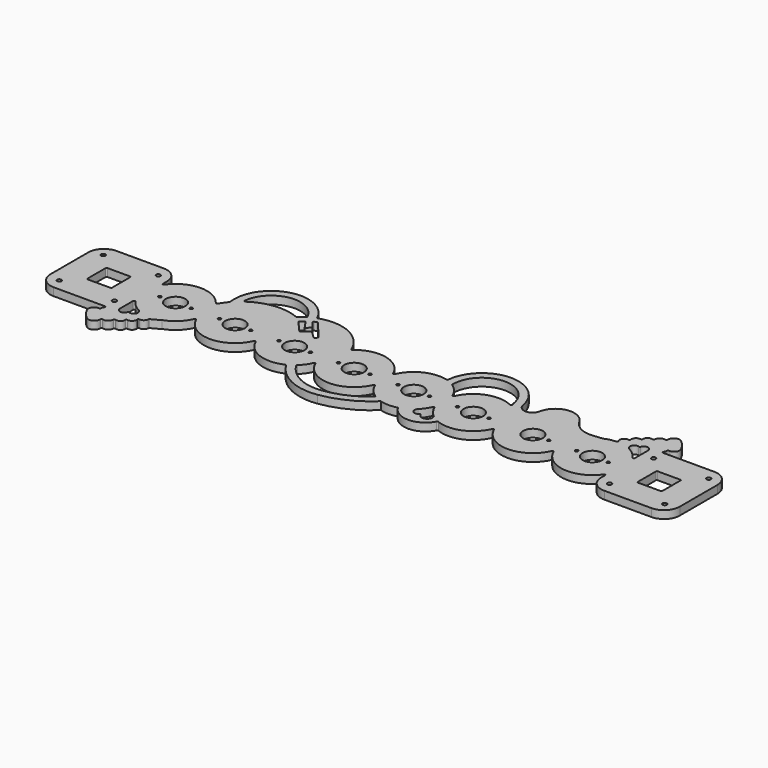
from build123d import *

# Parameters (mm, degrees)
F1_DEPTH  = 6.35
F2_R      = 25.4
F4_DEPTH  = 12.7
F6_DEPTH  = 12.7
F8_DEPTH  = 12.7
F10_DEPTH = 12.7
F12_DEPTH = 12.701
F14_DEPTH = 12.701
F16_D     = 6.7564
F18_D     = 31.75
F20_D     = 4.7625
F21_R     = 1.5875


# Not quite as in the source:
# - a feature names something its author has since deleted; it is built from what else it names


with BuildPart() as f1:
    # F0 (on Top) → F1 (new body, symmetric)
    with BuildSketch(Plane.XY):
        with BuildLine():
            Line((508, -63.5), (508, 63.5))
            Line((508, 63.5), (381, 63.5))
            Line((381, 63.5), (381, 24.5934442484))
            ThreePointArc((381, 24.5934442484), (385.7368884968, 12.7), (387.35, 0))
            ThreePointArc((387.35, 0), (385.7368884968, -12.7), (381, -24.5934442484))
            Line((381, -24.5934442484), (381, -63.5))
            Line((381, -63.5), (508, -63.5))
        make_face()
        with BuildLine():
            ThreePointArc((387.35, 0), (385.7368884968, 12.7), (381, 24.5934442484))
            Line((381, 24.5934442484), (381, 0))
            Line((381, 0), (387.35, 0))
        make_face()
        with BuildLine():
            Line((381, 0), (381, 24.5934442484))
            ThreePointArc((381, 24.5934442484), (332.0713380674, 50.6021895504), (288.4714285714, 16.4039924832))
            ThreePointArc((288.4714285714, 16.4039924832), (290.5078819786, 8.314101618), (291.1928571429, 0))
            ThreePointArc((291.1928571429, 0), (290.5078819786, -8.314101618), (288.4714285714, -16.4039924832))
            ThreePointArc((288.4714285714, -16.4039924832), (332.0713380674, -50.6021895504), (381, -24.5934442484))
            Line((381, -24.5934442484), (381, 0))
        make_face()
        with BuildLine():
            Line((387.35, 0), (381, 0))
            Line((381, 0), (381, -24.5934442484))
            ThreePointArc((381, -24.5934442484), (385.7368884968, -12.7), (387.35, 0))
        make_face()
        with BuildLine():
            ThreePointArc((288.4714285714, -16.4039924832), (285.75, 0), (288.4714285714, 16.4039924832))
            ThreePointArc((288.4714285714, 16.4039924832), (240.3928571429, 50.8), (192.3142857143, 16.4039924832))
            ThreePointArc((192.3142857143, 16.4039924832), (194.3507391214, 8.314101618), (195.0357142857, 0))
            ThreePointArc((195.0357142857, 0), (194.3507391214, -8.314101618), (192.3142857143, -16.4039924832))
            ThreePointArc((192.3142857143, -16.4039924832), (240.3928571429, -50.8), (288.4714285714, -16.4039924832))
        make_face()
        with BuildLine():
            ThreePointArc((291.1928571429, 0), (290.5078819786, 8.314101618), (288.4714285714, 16.4039924832))
            ThreePointArc((288.4714285714, 16.4039924832), (285.75, 0), (288.4714285714, -16.4039924832))
            ThreePointArc((288.4714285714, -16.4039924832), (290.5078819786, -8.314101618), (291.1928571429, 0))
        make_face()
        with BuildLine():
            ThreePointArc((192.3142857143, -16.4039924832), (189.5928571429, 0), (192.3142857143, 16.4039924832))
            ThreePointArc((192.3142857143, 16.4039924832), (144.2357142857, 50.8), (96.1571428571, 16.4039924832))
            ThreePointArc((96.1571428571, 16.4039924832), (98.1935962643, 8.314101618), (98.8785714286, 0))
            ThreePointArc((98.8785714286, 0), (98.1935962643, -8.314101618), (96.1571428571, -16.4039924832))
            ThreePointArc((96.1571428571, -16.4039924832), (144.2357142857, -50.8), (192.3142857143, -16.4039924832))
        make_face()
        with BuildLine():
            ThreePointArc((195.0357142857, 0), (194.3507391214, 8.314101618), (192.3142857143, 16.4039924832))
            ThreePointArc((192.3142857143, 16.4039924832), (189.5928571429, 0), (192.3142857143, -16.4039924832))
            ThreePointArc((192.3142857143, -16.4039924832), (194.3507391214, -8.314101618), (195.0357142857, 0))
        make_face()
        with BuildLine():
            ThreePointArc((96.1571428571, -16.4039924832), (93.4357142857, 0), (96.1571428571, 16.4039924832))
            ThreePointArc((96.1571428571, 16.4039924832), (48.0785714286, 50.8), (0, 16.4039924832))
            ThreePointArc((0, 16.4039924832), (2.0364534072, 8.314101618), (2.7214285714, 0))
            ThreePointArc((2.7214285714, 0), (2.0364534072, -8.314101618), (0, -16.4039924832))
            ThreePointArc((0, -16.4039924832), (48.0785714286, -50.8), (96.1571428571, -16.4039924832))
        make_face()
        with BuildLine():
            ThreePointArc((98.8785714286, 0), (98.1935962643, 8.314101618), (96.1571428571, 16.4039924832))
            ThreePointArc((96.1571428571, 16.4039924832), (93.4357142857, 0), (96.1571428571, -16.4039924832))
            ThreePointArc((96.1571428571, -16.4039924832), (98.1935962643, -8.314101618), (98.8785714286, 0))
        make_face()
        with BuildLine():
            ThreePointArc((0, -16.4039924832), (-2.7214285714, 0), (0, 16.4039924832))
            ThreePointArc((0, 16.4039924832), (-48.0785714286, 50.8), (-96.1571428571, 16.4039924832))
            ThreePointArc((-96.1571428571, 16.4039924832), (-94.12068945, 8.314101618), (-93.4357142857, 0))
            ThreePointArc((-93.4357142857, 0), (-94.12068945, -8.314101618), (-96.1571428571, -16.4039924832))
            ThreePointArc((-96.1571428571, -16.4039924832), (-48.0785714286, -50.8), (0, -16.4039924832))
        make_face()
        with BuildLine():
            ThreePointArc((2.7214285714, 0), (2.0364534072, 8.314101618), (0, 16.4039924832))
            ThreePointArc((0, 16.4039924832), (-2.7214285714, 0), (0, -16.4039924832))
            ThreePointArc((0, -16.4039924832), (2.0364534072, -8.314101618), (2.7214285714, 0))
        make_face()
        with BuildLine():
            ThreePointArc((-96.1571428571, -16.4039924832), (-98.8785714286, 0), (-96.1571428571, 16.4039924832))
            ThreePointArc((-96.1571428571, 16.4039924832), (-144.2357142857, 50.8), (-192.3142857143, 16.4039924832))
            ThreePointArc((-192.3142857143, 16.4039924832), (-190.2778323071, 8.314101618), (-189.5928571429, 0))
            ThreePointArc((-189.5928571429, 0), (-190.2778323071, -8.314101618), (-192.3142857143, -16.4039924832))
            ThreePointArc((-192.3142857143, -16.4039924832), (-144.2357142857, -50.8), (-96.1571428571, -16.4039924832))
        make_face()
        with BuildLine():
            ThreePointArc((-93.4357142857, 0), (-94.12068945, 8.314101618), (-96.1571428571, 16.4039924832))
            ThreePointArc((-96.1571428571, 16.4039924832), (-98.8785714286, 0), (-96.1571428571, -16.4039924832))
            ThreePointArc((-96.1571428571, -16.4039924832), (-94.12068945, -8.314101618), (-93.4357142857, 0))
        make_face()
        with BuildLine():
            ThreePointArc((-192.3142857143, -16.4039924832), (-195.0357142857, 0), (-192.3142857143, 16.4039924832))
            ThreePointArc((-192.3142857143, 16.4039924832), (-240.3928571429, 50.8), (-288.4714285714, 16.4039924832))
            ThreePointArc((-288.4714285714, 16.4039924832), (-286.4349751643, 8.314101618), (-285.75, 0))
            ThreePointArc((-285.75, 0), (-286.4349751643, -8.314101618), (-288.4714285714, -16.4039924832))
            ThreePointArc((-288.4714285714, -16.4039924832), (-240.3928571429, -50.8), (-192.3142857143, -16.4039924832))
        make_face()
        with BuildLine():
            ThreePointArc((-189.5928571429, 0), (-190.2778323071, 8.314101618), (-192.3142857143, 16.4039924832))
            ThreePointArc((-192.3142857143, 16.4039924832), (-195.0357142857, 0), (-192.3142857143, -16.4039924832))
            ThreePointArc((-192.3142857143, -16.4039924832), (-190.2778323071, -8.314101618), (-189.5928571429, 0))
        make_face()
        with BuildLine():
            ThreePointArc((-288.4714285714, -16.4039924832), (-291.1928571429, 0), (-288.4714285714, 16.4039924832))
            ThreePointArc((-288.4714285714, 16.4039924832), (-332.0713380674, 50.6021895504), (-381, 24.5934442484))
            Line((-381, 24.5934442484), (-381, 0))
            Line((-381, 0), (-381, -24.5934442484))
            ThreePointArc((-381, -24.5934442484), (-332.0713380674, -50.6021895504), (-288.4714285714, -16.4039924832))
        make_face()
        with BuildLine():
            ThreePointArc((-285.75, 0), (-286.4349751643, 8.314101618), (-288.4714285714, 16.4039924832))
            ThreePointArc((-288.4714285714, 16.4039924832), (-291.1928571429, 0), (-288.4714285714, -16.4039924832))
            ThreePointArc((-288.4714285714, -16.4039924832), (-286.4349751643, -8.314101618), (-285.75, 0))
        make_face()
        with BuildLine():
            ThreePointArc((-387.35, 0), (-385.7368884968, 12.7), (-381, 24.5934442484))
            Line((-381, 24.5934442484), (-381, 63.5))
            Line((-381, 63.5), (-508, 63.5))
            Line((-508, 63.5), (-508, -63.5))
            Line((-508, -63.5), (-381, -63.5))
            Line((-381, -63.5), (-381, -24.5934442484))
            ThreePointArc((-381, -24.5934442484), (-385.7368884968, -12.7), (-387.35, 0))
        make_face()
        with BuildLine():
            Line((-381, 0), (-381, 24.5934442484))
            ThreePointArc((-381, 24.5934442484), (-385.7368884968, 12.7), (-387.35, 0))
            Line((-387.35, 0), (-381, 0))
        make_face()
        with BuildLine():
            Line((-381, -24.5934442484), (-381, 0))
            Line((-381, 0), (-387.35, 0))
            ThreePointArc((-387.35, 0), (-385.7368884968, -12.7), (-381, -24.5934442484))
        make_face()
    extrude(amount=F1_DEPTH, both=True)

    # F2
    f2_edges = [f1.edges().sort_by_distance(p)[0] for p in [
        (508, -63.5, 0),
        (381, -63.5, 0),
        (508, 63.5, 0),
        (-508, -63.5, 0),
        (-508, 63.5, 0),
        (-381, 63.5, 0),
    ]]
    fillet(f2_edges, radius=F2_R)

    # F3 (on face) → F4 (join, through all)
    with BuildSketch(Plane.XY.offset(6.35)):
        with BuildLine():
            ThreePointArc((-367.2552444243, -56.6276222122), (-374.1276222122, -63.5), (-381, -56.6276222122))
            Line((-381, -56.6276222122), (-381, -63.5))
            Line((-381, -63.5), (-391.535417959, -63.5))
            Line((-391.535417959, -63.5), (-394.5178569695, -63.5))
            ThreePointArc((-394.5178569695, -63.5), (-399.2758099526, -67.1825538995), (-399.4201421738, -73.1974095106))
            ThreePointArc((-399.4201421738, -73.1974095106), (-409.2730898493, -75.0079193762), (-411.5812182426, -84.7563073039))
            ThreePointArc((-411.5812182426, -84.7563073039), (-405.652510141, -94.2560722227), (-397.9265391827, -102.3619025946))
            ThreePointArc((-397.9265391827, -102.3619025946), (-385.82556258, -103.1087125948), (-382.9926252365, -91.320335865))
            ThreePointArc((-382.9926252365, -91.320335865), (-371.9326843725, -91.8099168303), (-369.8217202848, -80.9422670357))
            ThreePointArc((-369.8217202848, -80.9422670357), (-359.9477437268, -83.4855580061), (-357.2103527895, -73.6636216957))
            ThreePointArc((-357.2103527895, -73.6636216957), (-347.2490954144, -72.7221806555), (-346.8697477111, -62.723728023))
            ThreePointArc((-346.8697477111, -62.723728023), (-336.1545012002, -61.4010311927), (-338.0772106471, -50.7770383898))
            ThreePointArc((-338.0772106471, -50.7770383898), (-349.2473790256, -49.187565155), (-359.791204809, -45.1717433694))
            ThreePointArc((-359.791204809, -45.1717433694), (-357.1773168684, -55.0343377987), (-367.2552444243, -56.6276222122))
        make_face()
        with BuildLine():
            ThreePointArc((-369.9145615101, -80.7840153575), (-369.867712705, -80.8628899897), (-369.8217202848, -80.9422670357))
            ThreePointArc((-369.8217202848, -80.9422670357), (-369.8686393277, -80.8634336098), (-369.9145615101, -80.7840153575))
        make_face(mode=Mode.SUBTRACT)
        with BuildLine():
            ThreePointArc((-359.3822419643, -71.2338685989), (-358.1586258109, -72.3256843374), (-357.2103527895, -73.6636216957))
            ThreePointArc((-357.2103527895, -73.6636216957), (-358.4281920915, -72.5666421893), (-359.3822419643, -71.2338685989))
        make_face(mode=Mode.SUBTRACT)
        with BuildLine():
            ThreePointArc((-347.9171395302, -61.664249748), (-347.3673959828, -62.1682383973), (-346.8697477111, -62.723728023))
            ThreePointArc((-346.8697477111, -62.723728023), (-347.4200709816, -62.2203124833), (-347.9171395302, -61.664249748))
        make_face(mode=Mode.SUBTRACT)
        with BuildLine():
            ThreePointArc((397.9265391827, 102.3619025946), (385.82556258, 103.1087125948), (382.9926252365, 91.320335865))
            ThreePointArc((382.9926252365, 91.320335865), (371.9326843725, 91.8099168303), (369.8217202848, 80.9422670357))
            ThreePointArc((369.8217202848, 80.9422670357), (359.9477437268, 83.4855580061), (357.2103527895, 73.6636216957))
            ThreePointArc((357.2103527895, 73.6636216957), (347.2490954144, 72.7221806555), (346.8697477111, 62.723728023))
            ThreePointArc((346.8697477111, 62.723728023), (336.1545012002, 61.4010311927), (338.0772106471, 50.7770383898))
            ThreePointArc((338.0772106471, 50.7770383898), (349.2473790256, 49.187565155), (359.791204809, 45.1717433694))
            ThreePointArc((359.791204809, 45.1717433694), (357.1773168684, 55.0343377987), (367.2552444243, 56.6276222122))
            ThreePointArc((367.2552444243, 56.6276222122), (374.1276222122, 63.5), (381, 56.6276222122))
            Line((381, 56.6276222122), (381, 63.5))
            Line((381, 63.5), (391.535417959, 63.5))
            Line((391.535417959, 63.5), (394.5178569695, 63.5))
            ThreePointArc((394.5178569695, 63.5), (399.2758099526, 67.1825538995), (399.4201421738, 73.1974095106))
            ThreePointArc((399.4201421738, 73.1974095106), (409.2730898493, 75.0079193762), (411.5812182426, 84.7563073039))
            ThreePointArc((411.5812182426, 84.7563073039), (405.652510141, 94.2560722227), (397.9265391827, 102.3619025946))
        make_face()
        with BuildLine():
            ThreePointArc((347.9171395302, 61.664249748), (347.3673959828, 62.1682383973), (346.8697477111, 62.723728023))
            ThreePointArc((346.8697477111, 62.723728023), (347.4200709816, 62.2203124833), (347.9171395302, 61.664249748))
        make_face(mode=Mode.SUBTRACT)
        with BuildLine():
            ThreePointArc((359.3822419643, 71.2338685989), (358.1586258109, 72.3256843374), (357.2103527895, 73.6636216957))
            ThreePointArc((357.2103527895, 73.6636216957), (358.4281920915, 72.5666421893), (359.3822419643, 71.2338685989))
        make_face(mode=Mode.SUBTRACT)
        with BuildLine():
            ThreePointArc((369.9145615101, 80.7840153575), (369.867712705, 80.8628899897), (369.8217202848, 80.9422670357))
            ThreePointArc((369.8217202848, 80.9422670357), (369.8686393277, 80.8634336098), (369.9145615101, 80.7840153575))
        make_face(mode=Mode.SUBTRACT)
        with BuildLine():
            ThreePointArc((-359.3822419643, -71.2338685989), (-358.4281920915, -72.5666421893), (-357.2103527895, -73.6636216957))
            ThreePointArc((-357.2103527895, -73.6636216957), (-358.1586258109, -72.3256843374), (-359.3822419643, -71.2338685989))
        make_face()
        with BuildLine():
            ThreePointArc((359.3822419643, 71.2338685989), (358.4281920915, 72.5666421893), (357.2103527895, 73.6636216957))
            ThreePointArc((357.2103527895, 73.6636216957), (358.1586258109, 72.3256843374), (359.3822419643, 71.2338685989))
        make_face()
        with BuildLine():
            Line((-394.5178569695, -63.5), (-391.535417959, -63.5))
            ThreePointArc((-391.535417959, -63.5), (-393.0266374642, -63.3393714806), (-394.5178569695, -63.5))
        make_face()
        with BuildLine():
            ThreePointArc((391.535417959, 63.5), (393.0266374642, 63.3393714806), (394.5178569695, 63.5))
            Line((394.5178569695, 63.5), (391.535417959, 63.5))
        make_face()
        with BuildLine():
            ThreePointArc((-347.9171395302, -61.664249748), (-347.4200709816, -62.2203124833), (-346.8697477111, -62.723728023))
            ThreePointArc((-346.8697477111, -62.723728023), (-347.3673959828, -62.1682383973), (-347.9171395302, -61.664249748))
        make_face()
        with BuildLine():
            ThreePointArc((347.9171395302, 61.664249748), (347.4200709816, 62.2203124833), (346.8697477111, 62.723728023))
            ThreePointArc((346.8697477111, 62.723728023), (347.3673959828, 62.1682383973), (347.9171395302, 61.664249748))
        make_face()
        with BuildLine():
            ThreePointArc((-369.9145615101, -80.7840153575), (-369.8686393277, -80.8634336098), (-369.8217202848, -80.9422670357))
            ThreePointArc((-369.8217202848, -80.9422670357), (-369.867712705, -80.8628899897), (-369.9145615101, -80.7840153575))
        make_face()
        with BuildLine():
            ThreePointArc((369.9145615101, 80.7840153575), (369.8686393277, 80.8634336098), (369.8217202848, 80.9422670357))
            ThreePointArc((369.8217202848, 80.9422670357), (369.867712705, 80.8628899897), (369.9145615101, 80.7840153575))
        make_face()
    extrude(amount=-F4_DEPTH)

    # F5 (on face) → F6 (join, through all)
    with BuildSketch(Plane.XY.offset(6.35)):
        with BuildLine():
            ThreePointArc((-96.1571428571, 16.4039924832), (-90.8173087367, 27.4597948519), (-82.9809490943, 36.9115704526))
            ThreePointArc((-82.9809490943, 36.9115704526), (-130.8422318474, 79.9787965588), (-193.3161765337, 64.4065588713))
            ThreePointArc((-193.3161765337, 64.4065588713), (-250.9099691425, 66.1809708183), (-294.4794948513, 28.4730152343))
            ThreePointArc((-294.4794948513, 28.4730152343), (-291.0733100427, 22.6386985165), (-288.4714285714, 16.4039924832))
            ThreePointArc((-288.4714285714, 16.4039924832), (-240.3928571429, 50.8), (-192.3142857143, 16.4039924832))
            ThreePointArc((-192.3142857143, 16.4039924832), (-144.2357142857, 50.8), (-96.1571428571, 16.4039924832))
        make_face()
    extrude(amount=-F6_DEPTH)

    # F7 (on face) → F8 (join, through all)
    with BuildSketch(Plane.XY.offset(6.35)):
        with BuildLine():
            ThreePointArc((83.7656706137, -36.1534362372), (83.9550454553, -35.9655197573), (84.1434308045, -35.7766113291))
            ThreePointArc((84.1434308045, -35.7766113291), (83.9508854481, -35.9613494249), (83.7656706137, -36.1534362372))
        make_face()
        with BuildLine():
            ThreePointArc((95.4040512443, -42.6564626396), (85.44939682, -46.8061350412), (83.7656706137, -36.1534362372))
            ThreePointArc((83.7656706137, -36.1534362372), (73.5641269958, -43.9445839374), (61.7353344999, -48.9298765828))
            ThreePointArc((61.7353344999, -48.9298765828), (93.6417910841, -66.7779790184), (124.1754629008, -46.6714721685))
            ThreePointArc((124.1754629008, -46.6714721685), (117.9002803183, -43.4405906699), (112.1334752911, -39.3711347504))
            ThreePointArc((112.1334752911, -39.3711347504), (105.8412183812, -51.5670772662), (95.4040512443, -42.6564626396))
        make_face()
    extrude(amount=-F8_DEPTH)

    # F9 (on face) → F10 (join, through all)
    with BuildSketch(Plane.XY.offset(6.35)):
        with BuildLine():
            ThreePointArc((-182.0226603491, 72.6526142414), (-176.3904420753, 75.6007470086), (-170.5094874455, 78.0148187015))
            ThreePointArc((-170.5094874455, 78.0148187015), (-170.5568162756, 78.1191984441), (-170.6041363364, 78.2235821624))
            ThreePointArc((-170.6041363364, 78.2235821624), (-239.6687234517, 111.4236270541), (-284.4827737452, 49.2636634883))
            ThreePointArc((-284.4827737452, 49.2636634883), (-284.3160508711, 46.355432178), (-284.237868795, 43.4434752013))
            ThreePointArc((-284.237868795, 43.4434752013), (-278.3846056881, 49.5054242977), (-271.9207238285, 54.9115455644))
            ThreePointArc((-271.9207238285, 54.9115455644), (-234.2322472862, 99.6404759723), (-182.171309974, 72.9804443578))
            ThreePointArc((-182.171309974, 72.9804443578), (-182.0969958744, 72.816524442), (-182.0226603491, 72.6526142414))
        make_face()
        with BuildLine():
            ThreePointArc((-334.7476987559, -56.2388105933), (-327.2196107482, -52.4224972156), (-320.0110904194, -48.032327342))
            ThreePointArc((-320.0110904194, -48.032327342), (-328.9197224231, -50.2236882765), (-338.0772106471, -50.7770383898))
            ThreePointArc((-338.0772106471, -50.7770383898), (-335.7944619736, -53.1311943645), (-334.7476987559, -56.2388105933))
        make_face()
        with BuildLine():
            ThreePointArc((-39.9105097608, -84.8183222938), (-0.2538043246, -72.4957892974), (33.819773991, -48.757837274))
            ThreePointArc((33.819773991, -48.757837274), (27.3119848215, -46.3615021401), (21.1912092832, -43.1011572567))
            ThreePointArc((21.1912092832, -43.1011572567), (-8.1953570474, -62.2113465581), (-41.7790417119, -72.2565314841))
            ThreePointArc((-41.7790417119, -72.2565314841), (-81.2411421561, -66.2360390268), (-110.4623167641, -39.0399610849))
            ThreePointArc((-110.4623167641, -39.0399610849), (-110.6709688482, -38.6772801775), (-110.8795096844, -38.3145352914))
            ThreePointArc((-110.8795096844, -38.3145352914), (-115.9430410517, -42.1919973605), (-121.4524997647, -45.404461632))
            ThreePointArc((-121.4524997647, -45.404461632), (-86.7550050708, -77.6766492884), (-39.9105097608, -84.8183222938))
        make_face()
        with BuildLine():
            ThreePointArc((220.0328796949, 52.2059049635), (234.7827122755, 66.4493455003), (253.2278236154, 57.4932845837))
            ThreePointArc((253.2278236154, 57.4932845837), (257.2682716347, 51.3634719412), (262.1682696159, 45.8963115253))
            ThreePointArc((262.1682696159, 45.8963115253), (269.1892727941, 41.8498081912), (275.4775033049, 36.7383669164))
            ThreePointArc((275.4775033049, 36.7383669164), (286.0308861222, 33.1603420388), (297.1163801208, 32.0254527403))
            ThreePointArc((297.1163801208, 32.0254527403), (305.6911453773, 40.3530803208), (315.9743973294, 46.4465776429))
            Line((315.9743973294, 46.4465776429), (302.9252466768, 45.2680818318))
            ThreePointArc((302.9252466768, 45.2680818318), (280.6885546193, 48.3226053131), (264.3191388693, 63.6797800325))
            ThreePointArc((264.3191388693, 63.6797800325), (232.7850053962, 78.9912419767), (207.5683948411, 54.6403694486))
            ThreePointArc((207.5683948411, 54.6403694486), (193.8953823203, 43.4936117915), (180.4476910094, 54.9111892957))
            ThreePointArc((180.4476910094, 54.9111892957), (118.9715717258, 103.7795589897), (63.1892609627, 48.5005882624))
            ThreePointArc((63.1892609627, 48.5005882624), (69.6241533484, 46.004650849), (75.6613232319, 42.6594866701))
            ThreePointArc((75.6613232319, 42.6594866701), (75.732863009, 44.2938758983), (75.78469518, 45.9290087722))
            ThreePointArc((75.78469518, 45.9290087722), (118.7840558259, 91.0419405521), (167.9370767614, 52.7261192423))
            ThreePointArc((167.9370767614, 52.7261192423), (169.453021528, 47.4048984585), (172.0412193393, 42.5146314663))
            ThreePointArc((172.0412193393, 42.5146314663), (177.5639598462, 38.3388581971), (182.4675977506, 33.450905619))
            ThreePointArc((182.4675977506, 33.450905619), (191.392806137, 30.9248271359), (200.6417233252, 31.6304815046))
            ThreePointArc((200.6417233252, 31.6304815046), (208.4349912366, 39.4884135756), (217.7450407232, 45.4721498439))
            ThreePointArc((217.7450407232, 45.4721498439), (219.1159556247, 48.7619041717), (220.0328796949, 52.2059049635))
        make_face()
        with BuildLine():
            ThreePointArc((192.3142857143, 16.4039924832), (195.8229595337, 24.3754841411), (200.6417233252, 31.6304815046))
            ThreePointArc((200.6417233252, 31.6304815046), (191.392806137, 30.9248271359), (182.4675977506, 33.450905619))
            ThreePointArc((182.4675977506, 33.450905619), (188.2246102464, 25.4089951033), (192.3142857143, 16.4039924832))
        make_face()
        with BuildLine():
            ThreePointArc((262.1682696159, 45.8963115253), (257.2682716347, 51.3634719412), (253.2278236154, 57.4932845837))
            ThreePointArc((253.2278236154, 57.4932845837), (234.7827122755, 66.4493455003), (220.0328796949, 52.2059049635))
            ThreePointArc((220.0328796949, 52.2059049635), (219.1159556247, 48.7619041717), (217.7450407232, 45.4721498439))
            ThreePointArc((217.7450407232, 45.4721498439), (239.9078309121, 50.7976844901), (262.1682696159, 45.8963115253))
        make_face()
        with BuildLine():
            ThreePointArc((297.1163801208, 32.0254527403), (286.0308861222, 33.1603420388), (275.4775033049, 36.7383669164))
            ThreePointArc((275.4775033049, 36.7383669164), (283.1994207272, 27.3539414728), (288.4714285714, 16.4039924832))
            ThreePointArc((288.4714285714, 16.4039924832), (292.1022395163, 24.5974914978), (297.1163801208, 32.0254527403))
        make_face()
    extrude(amount=-F10_DEPTH)

    # F11 (on face) → F12 (cut, through all)
    with BuildSketch(Plane.XY.offset(6.35)):
        Polygon((-135.6612890959, 37.8661416471), (-163.0945950747, 70.3279897571), (-169.1884696484, 67.3068240285), (-159.0773314238, 54.8510141671), (-166.0850197077, 47.2832992673), (-176.3016312942, 62.4161071867), (-183.3109110594, 56.2208108604), (-165.1418044918, 35.6645139039), (-153.1053036451, 45.8364859223), (-140.1678800292, 33.2382264791), align=None)
    extrude(amount=-F12_DEPTH, mode=Mode.SUBTRACT)

    # F13 (on face) → F14 (cut, through all)
    with BuildSketch(Plane.XY.offset(6.35)):
        with BuildLine():
            ThreePointArc((464.0896040747, 18.25625), (463.6246360898, 19.3787820151), (462.5021040747, 19.84375))
            Line((462.5021040747, 19.84375), (425.9896040747, 19.84375))
            ThreePointArc((425.9896040747, 19.84375), (424.8670720596, 19.3787820151), (424.4021040747, 18.25625))
            Line((424.4021040747, 18.25625), (424.4021040747, -18.25625))
            ThreePointArc((424.4021040747, -18.25625), (424.8670720596, -19.3787820151), (425.9896040747, -19.84375))
            Line((425.9896040747, -19.84375), (462.5021040747, -19.84375))
            ThreePointArc((462.5021040747, -19.84375), (463.6246360898, -19.3787820151), (464.0896040747, -18.25625))
            Line((464.0896040747, -18.25625), (464.0896040747, 18.25625))
        make_face()
        with BuildLine():
            ThreePointArc((-464.0896040747, -18.25625), (-463.6246360898, -19.3787820151), (-462.5021040747, -19.84375))
            Line((-462.5021040747, -19.84375), (-425.9896040747, -19.84375))
            ThreePointArc((-425.9896040747, -19.84375), (-424.8670720596, -19.3787820151), (-424.4021040747, -18.25625))
            Line((-424.4021040747, -18.25625), (-424.4021040747, 18.25625))
            ThreePointArc((-424.4021040747, 18.25625), (-424.8670720596, 19.3787820151), (-425.9896040747, 19.84375))
            Line((-425.9896040747, 19.84375), (-462.5021040747, 19.84375))
            ThreePointArc((-462.5021040747, 19.84375), (-463.6246360898, 19.3787820151), (-464.0896040747, 18.25625))
            Line((-464.0896040747, 18.25625), (-464.0896040747, -18.25625))
        make_face()
    extrude(amount=-F14_DEPTH, mode=Mode.SUBTRACT)

    # F16 (through all)
    with Locations(Plane.XY.offset(6.35)):
        with Locations((488.6958540747, 44.45), (488.6958540747, -44.45), (399.7958540747, -44.45), (399.7958540747, 44.45), (-488.6958540747, 44.45), (-399.7958540747, 44.45), (-399.7958540747, -44.45), (-488.6958540747, -44.45)):
            Hole(F16_D / 2)

    # F18 (through all)
    with Locations(Plane.XY.offset(6.35)):
        with Locations((-336.55, 0), (-240.3928571429, 0), (-48.0785714286, 0), (144.2357142857, 0), (240.3928571429, 0), (48.0785714286, 0), (336.55, 0), (-144.2357142857, 0)):
            Hole(F18_D / 2)

    # F20 (through all)
    with Locations(Plane.XY.offset(6.35)):
        with Locations((-361.95, 0), (-265.7928571429, 0), (-214.9928571429, 0), (-169.6357142857, 0), (-118.8357142857, 0), (-73.4785714286, 0), (-22.6785714286, 0), (22.6785714286, 0), (73.4785714286, 0), (118.8357142857, 0), (169.6357142857, 0), (265.7928571429, 0), (311.15, 0), (361.95, 0), (-311.15, 0)):
            Hole(F20_D / 2)

    # F21
    f21_edges = [f1.edges().sort_by_distance(p)[0] for p in [
        (-381, -24.593444, 0),
        (-382.992625, -91.320336, 0),
        (-369.82172, -80.942267, 0),
        (-357.210353, -73.663622, 0),
        (-346.869748, -62.723728, 0),
        (-334.747699, -56.238811, 0),
        (-367.255244, -56.627622, 0),
        (-394.517857, -63.5, 0),
        (-399.420142, -73.19741, 0),
        (-381, 24.593444, 0),
        (-294.479495, 28.473015, 0),
        (-288.471429, -16.403992, 0),
        (-192.314286, -16.403992, 0),
        (-121.4525, -45.404462, 0),
        (-110.87951, -38.314535, 0),
        (-96.157143, -16.403992, 0),
        (0, -16.403992, 0),
        (21.191209, -43.101157, 0),
        (96.157143, -16.403992, 0),
        (112.133475, -39.371135, 0),
        (95.404051, -42.656463, 0),
        (124.175463, -46.671472, 0),
        (192.314286, -16.403992, 0),
        (288.471429, -16.403992, 0),
        (381, -24.593444, 0),
        (381, 24.593444, 0),
        (338.077211, 50.777038, 0),
        (346.869748, 62.723728, 0),
        (357.210353, 73.663622, 0),
        (369.82172, 80.942267, 0),
        (382.992625, 91.320336, 0),
        (399.420142, 73.19741, 0),
        (394.517857, 63.5, 0),
        (367.255244, 56.627622, 0),
        (172.041219, 42.514631, 0),
        (96.157143, 16.403992, 0),
        (75.661323, 42.659487, 0),
        (63.189261, 48.500588, 0),
        (0, 16.403992, 0),
        (-82.980949, 36.91157, 0),
        (-170.604136, 78.223582, 0),
        (-193.316177, 64.406559, 0),
        (-182.17131, 72.980444, 0),
        (-271.920724, 54.911546, 0),
        (-165.141804, 35.664514, 0),
        (-176.301631, 62.416107, 0),
        (-166.08502, 47.283299, 0),
        (-159.077331, 54.851014, 0),
        (-169.18847, 67.306824, 0),
        (-163.094595, 70.32799, 0),
        (-135.661289, 37.866142, 0),
        (-140.16788, 33.238226, 0),
        (-153.105304, 45.836486, 0),
        (-183.310911, 56.220811, 0),
    ]]
    fillet(f21_edges, radius=F21_R)


solid = f1.part
